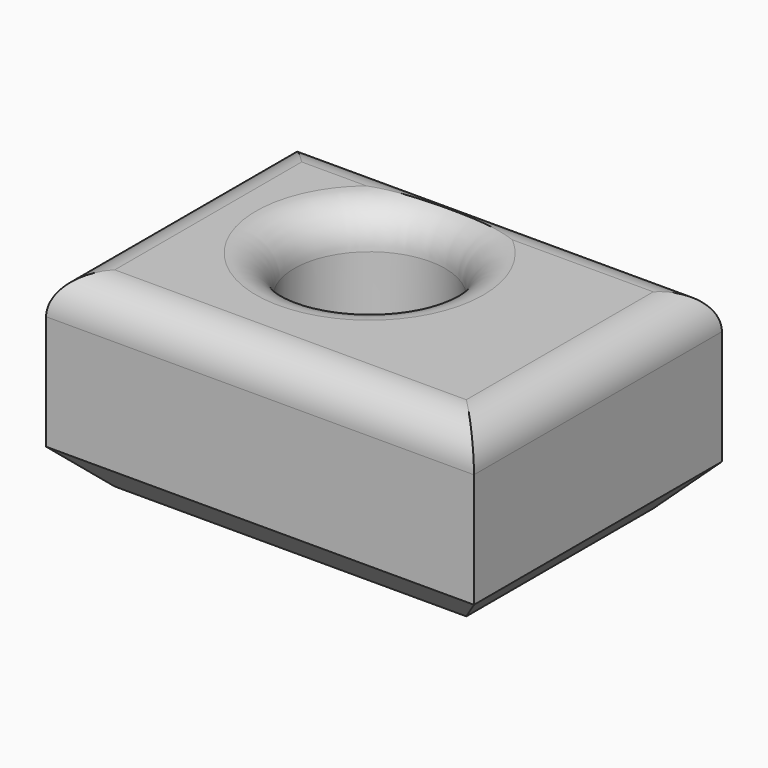
from build123d import *

# Parameters (mm, degrees)
F0_W        = 56.9857386872
F0_H        = 41.281120386
F0_R        = 10.0582455169
F1_DEPTH    = 25.4
F2_T1_DEPTH = 82.3857386872
F2_T3_DEPTH = 66.681120386
F3_T1_DEPTH = 83.114037845
F3_T3_DEPTH = 67.4094195437


# Not quite as in the source:
# - a fillet or chamfer that OpenCascade refuses, or shapes differently, is made with other operations: its cross-section is extruded or revolved along the edge and cut away or added


with BuildPart() as f1:
    # F0 (on Top) → F1 (new body)
    with BuildSketch(Plane.XY):
        with Locations((-38.084267173, -14.7667184938)):
            Rectangle(F0_W, F0_H)
        with Locations((-43.1615449488, -10.8050759882)):
            Circle(F0_R, mode=Mode.SUBTRACT)
    extrude(amount=F1_DEPTH)

    # F2: fillet of radius 5.08 on 5 edges, made by hand

    # F2_s2 → F2_t1 (cut)
    with BuildSketch(Plane.YZ.offset(-79.2771365166)):
        with BuildLine():
            ThreePointArc((5.8738416992, 20.32), (4.3859441476, 23.9121024484), (0.7938416992, 25.4))
            Line((0.7938416992, 25.4), (5.8738416992, 25.4))
            Line((5.8738416992, 25.4), (5.8738416992, 20.32))
        make_face()
        with BuildLine():
            ThreePointArc((-35.4072786868, 20.32), (-33.9193811352, 23.9121024484), (-30.3272786868, 25.4))
            Line((-30.3272786868, 25.4), (-35.4072786868, 25.4))
            Line((-35.4072786868, 25.4), (-35.4072786868, 20.32))
        make_face()
    extrude(amount=F2_T1_DEPTH, mode=Mode.SUBTRACT)

    # F2_s4 → F2_t3 (cut)
    with BuildSketch(Plane.XZ.offset(-18.5738416992)):
        with BuildLine():
            ThreePointArc((-66.5771365166, 20.32), (-65.089238965, 23.9121024484), (-61.4971365166, 25.4))
            Line((-61.4971365166, 25.4), (-66.5771365166, 25.4))
            Line((-66.5771365166, 25.4), (-66.5771365166, 20.32))
        make_face()
        with BuildLine():
            ThreePointArc((-9.5913978294, 20.32), (-11.0792953809, 23.9121024484), (-14.6713978294, 25.4))
            Line((-14.6713978294, 25.4), (-9.5913978294, 25.4))
            Line((-9.5913978294, 25.4), (-9.5913978294, 20.32))
        make_face()
    extrude(amount=F2_T3_DEPTH, mode=Mode.SUBTRACT)

    # F2_s5 → F2_t6 (revolve, cut)
    with BuildSketch(Plane.XZ.offset(10.8050759882)):
        with BuildLine():
            ThreePointArc((-33.103299432, 20.32), (-31.6154018804, 23.9121024484), (-28.023299432, 25.4))
            Line((-28.023299432, 25.4), (-33.103299432, 25.4))
            Line((-33.103299432, 25.4), (-33.103299432, 20.32))
        make_face()
    revolve(axis=Axis((-43.1615449488, -10.8050759882, 25.4), (0, 0, 1)), mode=Mode.SUBTRACT)

    # F3: chamfer of 5.08 on 5 edges, made by hand

    # F3_s2 → F3_t1 (cut)
    with BuildSketch(Plane.YZ.offset(-79.6412860954)):
        Polygon((5.8738416992, 5.08), (0.7938416992, 0), (5.8738416992, 0), align=None)
        Polygon((-30.3272786868, 0), (-35.4072786868, 5.08), (-35.4072786868, 0), align=None)
    extrude(amount=F3_T1_DEPTH, mode=Mode.SUBTRACT)

    # F3_s4 → F3_t3 (cut)
    with BuildSketch(Plane.XZ.offset(-18.9379912781)):
        Polygon((-61.4971365166, 0), (-66.5771365166, 5.08), (-66.5771365166, 0), align=None)
        Polygon((-14.6713978294, 0), (-9.5913978294, 5.08), (-9.5913978294, 0), align=None)
    extrude(amount=F3_T3_DEPTH, mode=Mode.SUBTRACT)

    # F3_s5 → F3_t6 (revolve, cut)
    with BuildSketch(Plane.XZ.offset(10.8050759882)):
        Polygon((-28.023299432, 0), (-33.103299432, 5.08), (-33.103299432, 0), align=None)
    revolve(axis=Axis((-43.1615449488, -10.8050759882, 0), (0, 0, 1)), mode=Mode.SUBTRACT)


solid = f1.part
